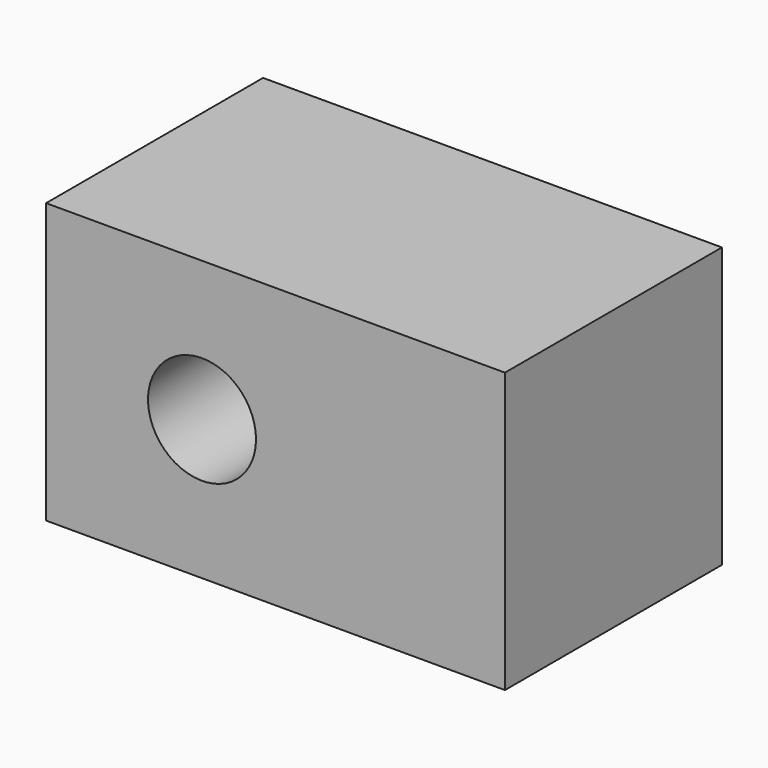
from build123d import *

# Parameters (mm, degrees)
F0_W     = 42.9752953351
F0_H     = 26.1746868491
F1_DEPTH = 25.4
F2_R     = 5.0570652765
F3_DEPTH = 25.401


# Not quite as in the source:
# - the program builds the solid bodies; features that only make, move or delete a surface that nothing else refers to are left out


with BuildPart() as f1:
    # F0 (on Front) → F1 (new body)
    with BuildSketch(Plane.XZ):
        with Locations((21.4876476675, 13.0873434246)):
            Rectangle(F0_W, F0_H)
    extrude(amount=-F1_DEPTH)

    # F2 (on face) → F3 (cut, through all)
    with BuildSketch(Plane.XZ):
        with Locations((14.6032562479, 13.0873434246)):
            Circle(F2_R)
    extrude(amount=-F3_DEPTH, mode=Mode.SUBTRACT)


solid = f1.part
